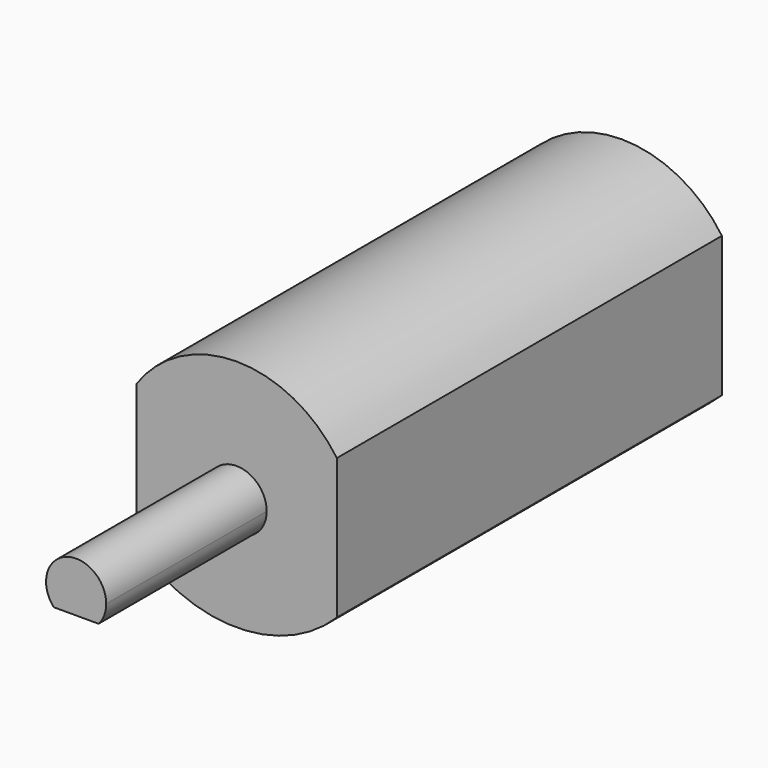
from build123d import *

# Parameters (mm, degrees)
F0_W     = 10
F0_H     = 7
F1_DEPTH = 24
F2_DEPTH = 34


with BuildPart() as f1:
    # F0 (on Front) → F1 (new body)
    with BuildSketch(Plane.XZ):
        with BuildLine():
            ThreePointArc((-6.6169165431, 2.8701706491), (-11.6169165431, 5.485347467), (-16.6169165431, 2.8701706491))
            Line((-16.6169165431, 2.8701706491), (-6.6169165431, 2.8701706491))
        make_face()
        with BuildLine():
            Line((-6.6169165431, -4.1298293509), (-16.6169165431, -4.1298293509))
            ThreePointArc((-16.6169165431, -4.1298293509), (-11.6169165431, -6.1927828871), (-6.6169165431, -4.1298293509))
        make_face()
        with Locations((-11.6169165431, -0.6298293509)):
            Rectangle(F0_W, F0_H)
        with BuildLine():
            ThreePointArc((-12.7349732604, -1.6020070586), (-12.1521337532, 0.7992321504), (-10.1169165431, -0.6020324705))
            ThreePointArc((-10.1169165431, -0.6020324705), (-10.2156519221, -1.1372496806), (-10.4988598258, -1.6020070586))
            ThreePointArc((-10.4988598258, -1.6020070586), (-11.6169165431, -2.1020324705), (-12.7349732604, -1.6020070586))
        make_face(mode=Mode.SUBTRACT)
    extrude(amount=F1_DEPTH)

    # F0 (on Front) → F2 (join)
    with BuildSketch(Plane.XZ):
        with BuildLine():
            ThreePointArc((-10.4988598258, -1.6020070586), (-10.2156519221, -1.1372496806), (-10.1169165431, -0.6020324705))
            ThreePointArc((-10.1169165431, -0.6020324705), (-12.1521337532, 0.7992321504), (-12.7349732604, -1.6020070586))
            Line((-12.7349732604, -1.6020070586), (-11.6097875087, -1.6020070586))
            Line((-11.6097875087, -1.6020070586), (-10.4988598258, -1.6020070586))
        make_face()
    extrude(amount=F2_DEPTH)


solid = f1.part
